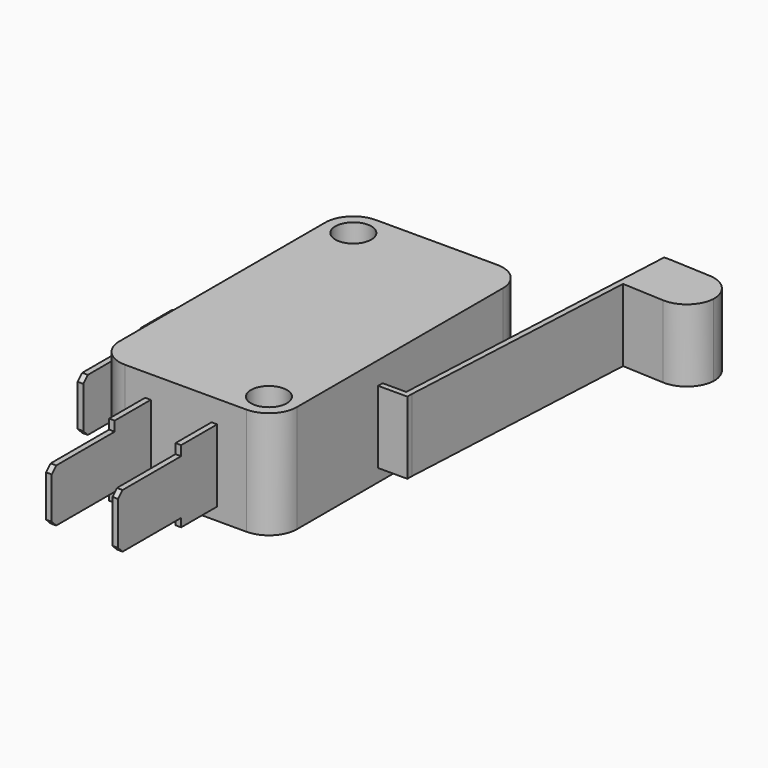
from build123d import *

# Parameters (mm, degrees)
F0_W         = 15.79
F0_H         = 27.86
F1_DEPTH     = 9.555
F2_R         = 2.5
F3_R         = 1.6
F4_DEPTH     = 25
F5_W         = 0.5
F5_H         = 6.4308560686
F6_DEPTH     = 4
F7_W         = 0.5
F7_H         = 4.7
F7_H_2       = 4.8242840722
F8_DEPTH     = 7
F9_SIZE      = 0.5
F10_W        = 0.5
F10_H        = 6.4308560686
F11_DEPTH    = 2.5
F12_W        = 0.5
F12_H        = 6.4308560686
F13_DEPTH    = 3
F14_W        = 0.5
F14_H        = 4.7
F15_DEPTH    = 7
F16_SIZE     = 0.5
F17_W        = 0.5
F17_H        = 6.4308560686
F18_DEPTH    = 2.6
F20_DEPTH    = 6.4308560686
F21_W        = 4.9
F21_H        = 6.4308560686
F22_DEPTH    = 6.2
F23_T1_DEPTH = 18.9308560686


# Not quite as in the source:
# - a fillet or chamfer that OpenCascade refuses, or shapes differently, is made with other operations: its cross-section is extruded or revolved along the edge and cut away or added


with BuildPart() as f1:
    # F0 (on Top) → F1 (new body)
    with BuildSketch(Plane.XY):
        Rectangle(F0_W, F0_H)
    extrude(amount=F1_DEPTH)

    # F2
    f2_edges = [f1.edges().sort_by_distance(p)[0] for p in [
        (-7.895, 13.93, 4.7775),
        (7.895, 13.93, 4.7775),
        (-7.895, -13.93, 4.7775),
        (7.895, -13.93, 4.7775),
    ]]
    fillet(f2_edges, radius=F2_R)

    # F3 (on face) → F4 (cut)
    with BuildSketch(Plane.XY.offset(9.555)):
        with Locations((-5.395, 11.43)):
            Circle(F3_R)
        with Locations((5.395, -11.43)):
            Circle(F3_R)
    extrude(amount=-F4_DEPTH, mode=Mode.SUBTRACT)

    # F5 (on face) → F6 (join)
    with BuildSketch(Plane.XZ.offset(13.93)):
        with Locations((-3.355, 4.3395719657)):
            Rectangle(F5_W, F5_H)
        with Locations((2.545, 4.3395719657)):
            Rectangle(F5_W, F5_H)
    extrude(amount=F6_DEPTH)

    # F7 (on face) → F8 (join)
    with BuildSketch(Plane.XZ.offset(17.93)):
        with Locations((-3.355, 4.3395719657)):
            Rectangle(F7_W, F7_H)
        with Locations((2.545, 4.2774299296)):
            Rectangle(F7_W, F7_H_2)
    extrude(amount=F8_DEPTH)

    # F9
    f9_edges = [f1.edges().sort_by_distance(p)[0] for p in [
        (-3.355, -24.93, 6.689572),
        (2.545, -24.93, 6.689572),
        (2.545, -24.93, 1.865288),
        (-3.355, -24.93, 1.989572),
    ]]
    chamfer(f9_edges, length=F9_SIZE)

    # F10 (on face) → F11 (join)
    with BuildSketch(Plane(origin=(-7.895, 0, 0), x_dir=(0, -1, 0), z_dir=(-1, 0, 0))):
        with Locations((2.68, 4.3395719657)):
            Rectangle(F10_W, F10_H)
    extrude(amount=F11_DEPTH)

    # F12 (on face) → F13 (join)
    with BuildSketch(Plane.XZ.offset(2.93)):
        with Locations((-10.145, 4.3395719657)):
            Rectangle(F12_W, F12_H)
    extrude(amount=F13_DEPTH)

    # F14 (on face) → F15 (join)
    with BuildSketch(Plane.XZ.offset(5.93)):
        with Locations((-10.145, 4.3395719657)):
            Rectangle(F14_W, F14_H)
    extrude(amount=F15_DEPTH)

    # F16
    f16_edges = [f1.edges().sort_by_distance(p)[0] for p in [
        (-10.145, -12.93, 6.689572),
        (-10.145, -12.93, 1.989572),
    ]]
    chamfer(f16_edges, length=F16_SIZE)

    # F17 (on face) → F18 (join)
    with BuildSketch(Plane.YZ.offset(7.895)):
        with Locations((-2.18, 4.3395719657)):
            Rectangle(F17_W, F17_H)
    extrude(amount=F18_DEPTH)

    # F19 (on face) → F20 (join, through all)
    with BuildSketch(Plane.XY.offset(7.555)):
        Polygon((11.3426885902, 25.0363132727), (9.9943753924, -1.93), (10.495, -1.93), (11.8433131978, 25.0363132727), align=None)
    extrude(amount=-F20_DEPTH)

    # F21 (on face) → F22 (join)
    with BuildSketch(Plane(origin=(10.5650872021, -0.528253394, 0), x_dir=(0.0499375258, 0.9987523434, 0), z_dir=(0.9987523434, -0.0499375258, 0))):
        with Locations((23.1465023109, 4.3395719657)):
            Rectangle(F21_W, F21_H)
    extrude(amount=F22_DEPTH)

    # F23: fillet of radius 2.5 on 2 edges, made by hand

    # F23_s2 → F23_t1 (cut)
    with BuildSketch(Plane.XY.offset(-5.1258560686)):
        with BuildLine():
            ThreePointArc((15.2940029919, 19.9576579442), (17.0961302855, 20.600699508), (17.9157276651, 22.3296949882))
            Line((17.9157276651, 22.3296949882), (17.7908838505, 19.8328141296))
            Line((17.7908838505, 19.8328141296), (15.2940029919, 19.9576579442))
        make_face()
        with BuildLine():
            ThreePointArc((15.5386968685, 24.8515444271), (17.2676923487, 24.0319470475), (17.9107339125, 22.2298197539))
            Line((17.9107339125, 22.2298197539), (18.0355777271, 24.7267006124))
            Line((18.0355777271, 24.7267006124), (15.5386968685, 24.8515444271))
        make_face()
    extrude(amount=F23_T1_DEPTH, mode=Mode.SUBTRACT)


solid = f1.part
